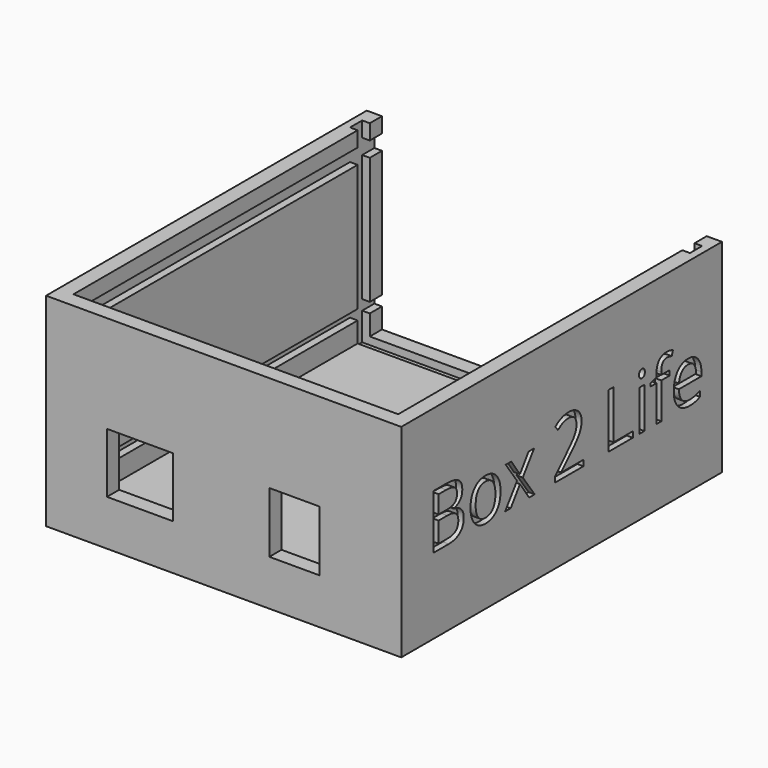
from build123d import *

# Parameters (mm, degrees)
F1_DEPTH      = 67
F2_W          = 70
F2_H          = 40
F2_W_2        = 13
F2_H_2        = 11.8
F2_W_3        = 9.93
F2_H_3        = 11.94
F3_DEPTH      = 3
F5_DEPTH      = 9
F7_W          = 3
F7_H          = 38.5
F8_DEPTH      = 1.5
F10_W         = 3
F10_H         = 38.5
F11_DEPTH     = 1.5
F12_W         = 65.4999999478
F12_H         = 3
F13_DEPTH     = 1.5
F14_TEXT_SIZE = 15.0348409079
F15_DEPTH     = 1.2


# Not quite as in the source:
# - Text() gives the source's letters only with a copy of the font that has no kerning and outlines rounded to 1/6400 em; it was checked with that copy


with BuildPart() as f1:
    # F0 (on Front) → F1 (new body)
    with BuildSketch(Plane.XZ):
        Polygon((0, 40), (0, 0), (70, 0), (70, 40), (66.9999999739, 40), (66.9999999739, 37), (68.4999999739, 37), (68.4999999739, 34), (66.9999999739, 34), (66.9999999739, 18.0000000261), (55.5400000261, 18.0000000261), (55.5400000261, 9.0000000261), (57.0400000261, 9.0000000261), (57.0400000261, 7.0000000261), (55.5400000261, 7.0000000261), (55.5400000261, 3.0000000261), (3.0000000261, 3.0000000261), (3.0000000261, 7.0000000261), (1.5000000261, 7.0000000261), (1.5000000261, 9.0000000261), (3.0000000261, 9.0000000261), (3.0000000261, 34), (1.5000000261, 34), (1.5000000261, 37), (3.0000000261, 37), (3.0000000261, 40), align=None)
    extrude(amount=-F1_DEPTH)

    # F2 (on face) → F3 (join)
    with BuildSketch(Plane.XZ):
        with Locations((35, 20)):
            Rectangle(F2_W, F2_H)
        with Locations((18.5000000261, 14.9000000261)):
            Rectangle(F2_W_2, F2_H_2, mode=Mode.SUBTRACT)
        with Locations((48.9650000261, 14.9700000261)):
            Rectangle(F2_W_3, F2_H_3, mode=Mode.SUBTRACT)
    extrude(amount=F3_DEPTH)

    # F4 (on face) → F5 (join)
    with BuildSketch(Plane(origin=(0, 67, 0), x_dir=(-1, 0, 0), z_dir=(0, 1, 0))):
        Polygon((-70, 40), (-70, 0), (0, 0), (0, 40), (-3.0000000261, 40), (-3.0000000261, 37), (-1.5000000261, 37), (-1.5000000261, 34), (-3.0000000261, 34), (-3.0000000261, 9.0000000261), (-1.5000000261, 9.0000000261), (-1.5000000261, 7.0000000261), (-3.0000000261, 7.0000000261), (-3.0000000261, 3.0000000261), (-55.5400000261, 3.0000000261), (-66.9999999739, 3.0000000261), (-66.9999999739, 18.0000000261), (-66.9999999739, 34), (-68.4999999739, 34), (-68.4999999739, 37), (-66.9999999739, 37), (-66.9999999739, 40), align=None)
    extrude(amount=F5_DEPTH)

    # F7 (on offset) → F8 (cut)
    with BuildSketch(Plane(origin=(66.9999999739, 0, 0), x_dir=(0, -1, 0), z_dir=(-1, 0, 0))):
        with Locations((-71.5, 20.75)):
            Rectangle(F7_W, F7_H)
    extrude(amount=-F8_DEPTH, mode=Mode.SUBTRACT)

    # F10 (on offset) → F11 (cut)
    with BuildSketch(Plane.YZ.offset(3.0000000261)):
        with Locations((71.5, 20.75)):
            Rectangle(F10_W, F10_H)
    extrude(amount=-F11_DEPTH, mode=Mode.SUBTRACT)

    # F12 (on face) → F13 (cut)
    with BuildSketch(Plane.XY.offset(3.0000000261)):
        with Locations((35.75, 71.5)):
            Rectangle(F12_W, F12_H)
    extrude(amount=-F13_DEPTH, mode=Mode.SUBTRACT)

    # F14 (on face) → F15 (cut)
    with BuildSketch(Plane.YZ.offset(70)):
        with Locations((3.4793014638, 14.9210998788)):
            Text('Box 2 Life', F14_TEXT_SIZE, font='Open Sans', text_align=(TextAlign.LEFT, TextAlign.BOTTOM))
    extrude(amount=-F15_DEPTH, mode=Mode.SUBTRACT)


solid = f1.part
